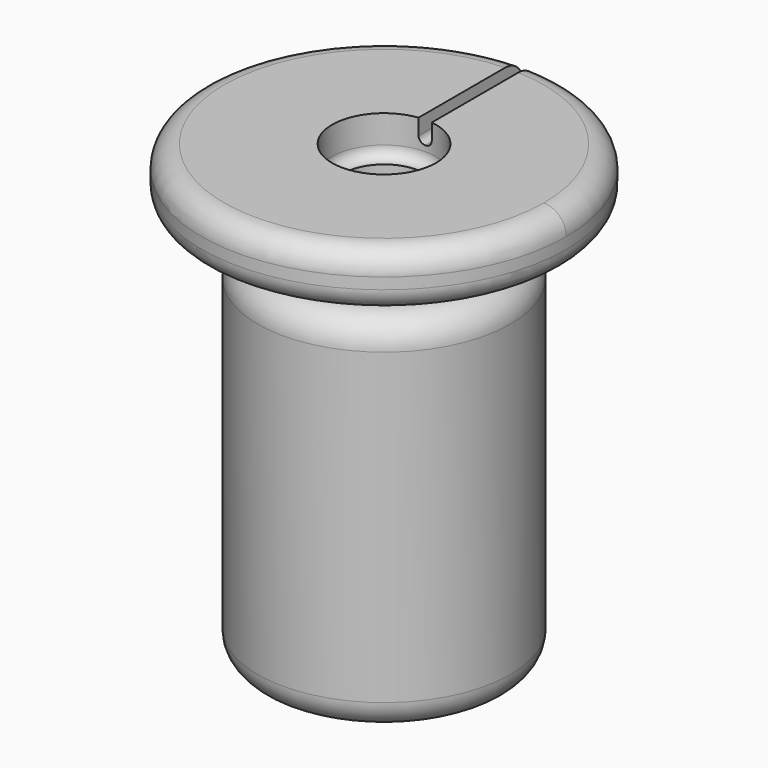
from build123d import *

# Parameters (mm, degrees)
F0_R      = 45
F1_DEPTH  = 130
F2_R      = 10
F3_T      = -2.5
F4_R      = 17.5
F5_DEPTH  = 25
F9_R      = 8
F10_R     = 10
F12_W     = 4.7
F12_H     = 8
F13_DEPTH = 100
F14_R     = 2.3
F15_R     = 3.99999


# Not quite as in the source:
# - a fillet or chamfer that OpenCascade refuses, or shapes differently, is made with other operations: its cross-section is extruded or revolved along the edge and cut away or added
# - a fillet or chamfer is up to 0.001 mm smaller than in the source, because OpenCascade refuses the exact size
# - a feature names something its author has since deleted; it is built from what else it names


with BuildPart() as f1:
    # F0 (on Top) → F1 (new body)
    with BuildSketch(Plane.XY):
        Circle(F0_R)
    extrude(amount=F1_DEPTH)

    # F2
    f2_edges = [f1.edges().sort_by_distance(p)[0] for p in [
        (-45, 0, 0),
        (-45, 0, 130),
    ]]
    fillet(f2_edges, radius=F2_R)

    # F3: a shell. OpenCascade refuses it in one call, so the cavity is built on its own and cut out:
    # the body offset inwards by the wall thickness, plus a prism from it out through each open face.
    f3_core = offset(f1.part, amount=F3_T, mode=Mode.PRIVATE)
    f3_exits = [f3_core.faces().sort_by_distance(p)[0] for p in [
        (0, 0, 2.5),
    ]]
    add(f3_core, mode=Mode.SUBTRACT)
    extrude(f3_exits, amount=-F3_T, mode=Mode.SUBTRACT)

    # F4 (on face) → F5 (cut)
    with BuildSketch(Plane.XY.offset(130)):
        Circle(F4_R)
    extrude(amount=-F5_DEPTH, mode=Mode.SUBTRACT)


with BuildPart() as f8:
    # F7 (on Front) → F8 (revolve)
    with BuildSketch(Plane.XZ):
        Polygon((21, 142), (65, 142), (65, 162), (18.5, 162), (18.5, 148), (14.5, 148), (14.5, 126), (17.4, 126), (17.4, 130), (21, 130), align=None)
    revolve(axis=Axis((0, 0, 127.8810352087), (0, 0, 1)))

    # F9
    f9_edges = [f8.edges().sort_by_distance(p)[0] for p in [
        (-65, 0, 142),
        (-65, 0, 162),
    ]]
    fillet(f9_edges, radius=F9_R)

    # F10
    f10_edges = [f8.edges().sort_by_distance(p)[0] for p in [
        (-21, 0, 142),
    ]]
    fillet(f10_edges, radius=F10_R)

    # F11: chamfer of 0.3 x 2 on 1 edges, made by hand

    # F11_s1 → F11_t2 (revolve, cut)
    with BuildSketch(Plane.XZ):
        Polygon((17.4, 128), (17.1, 126), (17.4, 126), align=None)
    revolve(axis=Axis((0, 0, 126), (0, 0, 1)), mode=Mode.SUBTRACT)

    # F12 (on Front) → F13 (cut)
    with BuildSketch(Plane.XZ):
        with Locations((0, 158)):
            Rectangle(F12_W, F12_H)
    extrude(amount=-F13_DEPTH, mode=Mode.SUBTRACT)

    # F14
    f14_edges = [f8.edges().sort_by_distance(p)[0] for p in [
        (-2.35, 41.653821, 154),
        (2.35, 41.653821, 154),
    ]]
    fillet(f14_edges, radius=F14_R)

    # F15 (radius 4 in the source; OpenCascade refuses exactly that, so slightly less here)
    f15_edges = [f8.edges().sort_by_distance(p)[0] for p in [
        (-18.5, 0, 148),
    ]]
    fillet(f15_edges, radius=F15_R)


solid = Compound([f1.part, f8.part])
